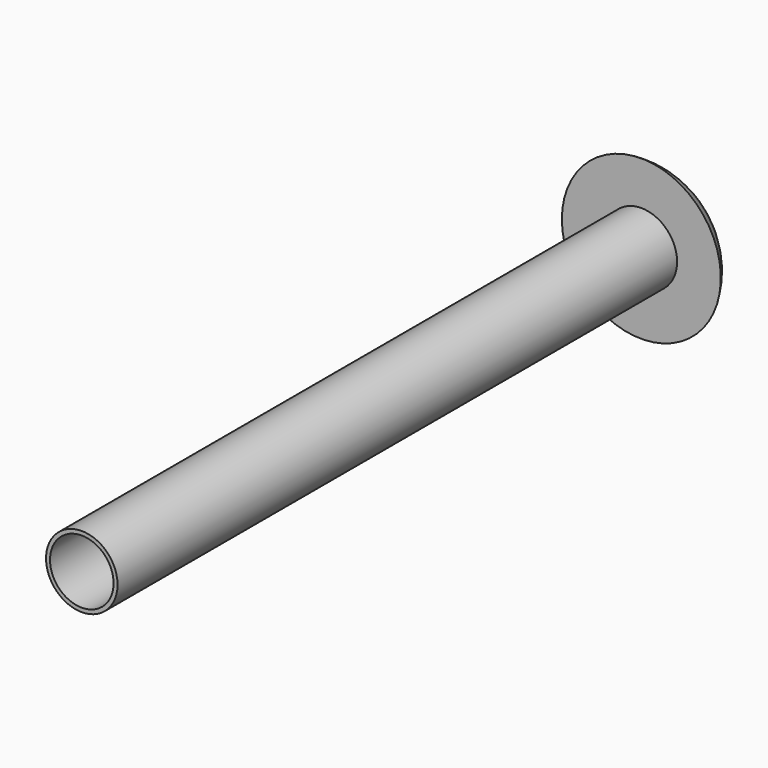
from build123d import *

# Parameters (mm, degrees)
F0_R     = 4.5
F1_DEPTH = 88
F2_R     = 4
F3_DEPTH = 25
F4_R     = 10
F4_R_2   = 4.5
F5_DEPTH = 5


# Not quite as in the source:
# - a fillet or chamfer that OpenCascade refuses, or shapes differently, is made with other operations: its cross-section is extruded or revolved along the edge and cut away or added


with BuildPart() as f1:
    # F0 (on Front) → F1 (new body)
    with BuildSketch(Plane.XZ):
        Circle(F0_R)
    extrude(amount=F1_DEPTH)

    # F2 (on face) → F3 (cut)
    with BuildSketch(Plane.XZ.offset(88)):
        Circle(F2_R)
    extrude(amount=-F3_DEPTH, mode=Mode.SUBTRACT)

    # F4 (on face) → F5 (join)
    with BuildSketch(Plane(origin=(0, 0, 0), x_dir=(-1, 0, 0), z_dir=(0, 1, 0))):
        Circle(F4_R)
        Circle(F4_R_2, mode=Mode.SUBTRACT)
        Circle(F4_R_2)
    extrude(amount=F5_DEPTH)

    # F6: fillet of radius 10 on 1 edges, made by hand

    # F6_s1 → F6_t2 (revolve, cut)
    with BuildSketch(Plane.XY):
        with BuildLine():
            ThreePointArc((-10, 0), (-6.3397459622, 3.6602540378), (-1.3397459622, 5))
            Line((-1.3397459622, 5), (-10, 5))
            Line((-10, 5), (-10, 0))
        make_face()
    revolve(axis=Axis((0, 5, 0), (0, 1, 0)), mode=Mode.SUBTRACT)


solid = f1.part
